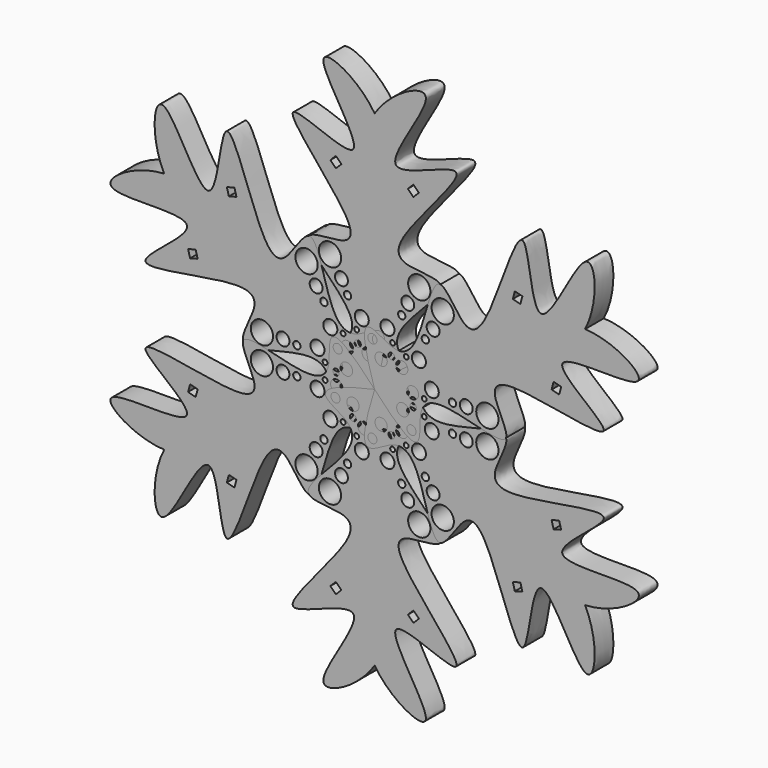
from build123d import *

# Parameters (mm, degrees)
F0_R     = 1.1694827394
F0_R_2   = 1.5672074123
F0_R_3   = 0.8059186056
F0_R_4   = 1.5208223034
F0_R_5   = 0.6193262095
F0_R_6   = 0.9345024276
F0_R_7   = 1.7945114962
F0_R_8   = 1.6498807188
F0_R_9   = 2.8514445583
F1_DEPTH = 6
F3_COUNT = 6


with BuildPart() as f1:
    # F0 (on Front) → F1 (new body)
    with BuildSketch(Plane.XZ):
        with BuildLine():
            add(Edge.make_bspline(
                [(0, 62.230002135), (4.0806569159, 68.6424598098), (22.4575884825, 77.8707801419), (-5.4515225932, 43.3617108178), (32.8949814803, 64.4366837068), (4.9583984864, 37.0325187292), (6.1875576647, 29.6267848256), (23.0235108368, 31.1980334768), (6.7059785993, 18.000598893), (3.5606618896, 8.1418871821), (19.978202205, 4.4237445395), (0, 0)],
                knots=[0, 0, 0, 0, 0.1198038554, 0.2544732475, 0.3752865526, 0.5236201237, 0.5959059312, 0.6891368853, 0.8051423582, 0.8943072746, 1, 1, 1, 1], degree=3))
            add(Edge.make_bspline(
                [(0, 62.230002135), (-4.0806569159, 68.6424598098), (-22.4575884825, 77.8707801419), (5.4515225932, 43.3617108178), (-32.8949814803, 64.4366837068), (-4.9583984864, 37.0325187292), (-6.1875576647, 29.6267848256), (-23.0235108368, 31.1980334768), (-6.7059785993, 18.000598893), (-3.5606618896, 8.1418871821), (-19.978202205, 4.4237445395), (0, 0)],
                knots=[0, 0, 0, 0, 0.1198038554, 0.2544732475, 0.3752865526, 0.5236201237, 0.5959059312, 0.6891368853, 0.8051423582, 0.8943072746, 1, 1, 1, 1], degree=3))
        make_face()
        with Locations((-10.0128995255, 5.1275761798)):
            Circle(F0_R, mode=Mode.SUBTRACT)
        with Locations((-5.5380342528, 5.1275761798)):
            Circle(F0_R_2, mode=Mode.SUBTRACT)
        with Locations((-5.5380342528, 8.2020899281)):
            Circle(F0_R_3, mode=Mode.SUBTRACT)
        with Locations((-2.759429859, 9.6626663581)):
            Circle(F0_R_4, mode=Mode.SUBTRACT)
        with Locations((-4.6076229773, 11.9972834364)):
            Circle(F0_R_5, mode=Mode.SUBTRACT)
        with Locations((-6.9331889972, 18.9996156842)):
            Circle(F0_R_6, mode=Mode.SUBTRACT)
        with Locations((-3.2929691952, 14.9980662391)):
            Circle(F0_R_7, mode=Mode.SUBTRACT)
        with Locations((-8.4949843585, 22.2008563578)):
            Circle(F0_R_8, mode=Mode.SUBTRACT)
        with Locations((-11.4294532686, 26.7359465361)):
            Circle(F0_R_9, mode=Mode.SUBTRACT)
        with Locations((2.759429859, 9.6626663581)):
            Circle(F0_R_4, mode=Mode.SUBTRACT)
        with Locations((5.5380342528, 5.1275761798)):
            Circle(F0_R_2, mode=Mode.SUBTRACT)
        with Locations((5.5380342528, 8.2020899281)):
            Circle(F0_R_3, mode=Mode.SUBTRACT)
        with Locations((10.0128995255, 5.1275761798)):
            Circle(F0_R, mode=Mode.SUBTRACT)
        with Locations((4.6076229773, 11.9972834364)):
            Circle(F0_R_5, mode=Mode.SUBTRACT)
        with Locations((3.2929691952, 14.9980662391)):
            Circle(F0_R_7, mode=Mode.SUBTRACT)
        with Locations((6.9331889972, 18.9996156842)):
            Circle(F0_R_6, mode=Mode.SUBTRACT)
        with Locations((8.4949843585, 22.2008563578)):
            Circle(F0_R_8, mode=Mode.SUBTRACT)
        with Locations((11.4294532686, 26.7359465361)):
            Circle(F0_R_9, mode=Mode.SUBTRACT)
        Polygon((-11.3427988253, 48.0167749338), (-9.928585263, 49.4309884962), (-8.5143717006, 48.0167749338), (-9.928585263, 46.6025613714), align=None, mode=Mode.SUBTRACT)
        Polygon((8.5143717006, 48.0167749338), (9.928585263, 49.4309884962), (11.3427988253, 48.0167749338), (9.928585263, 46.6025613714), align=None, mode=Mode.SUBTRACT)
    extrude(amount=F1_DEPTH)


with BuildPart() as f3_1:
    # F3: instance of F1
    add(f1.part.rotate(Axis((0, -29.3043628335, 0), (0, -1, 0)), 1 * 360 / F3_COUNT))


with BuildPart() as f3_2:
    # F3: instance of F1
    add(f1.part.rotate(Axis((0, -29.3043628335, 0), (0, -1, 0)), 2 * 360 / F3_COUNT))


with BuildPart() as f3_3:
    # F3: instance of F1
    add(f1.part.rotate(Axis((0, -29.3043628335, 0), (0, -1, 0)), 3 * 360 / F3_COUNT))


with BuildPart() as f3_4:
    # F3: instance of F1
    add(f1.part.rotate(Axis((0, -29.3043628335, 0), (0, -1, 0)), 4 * 360 / F3_COUNT))


with BuildPart() as f3_5:
    # F3: instance of F1
    add(f1.part.rotate(Axis((0, -29.3043628335, 0), (0, -1, 0)), 5 * 360 / F3_COUNT))


solid = Compound([f1.part, f3_1.part, f3_2.part, f3_3.part, f3_4.part, f3_5.part])
